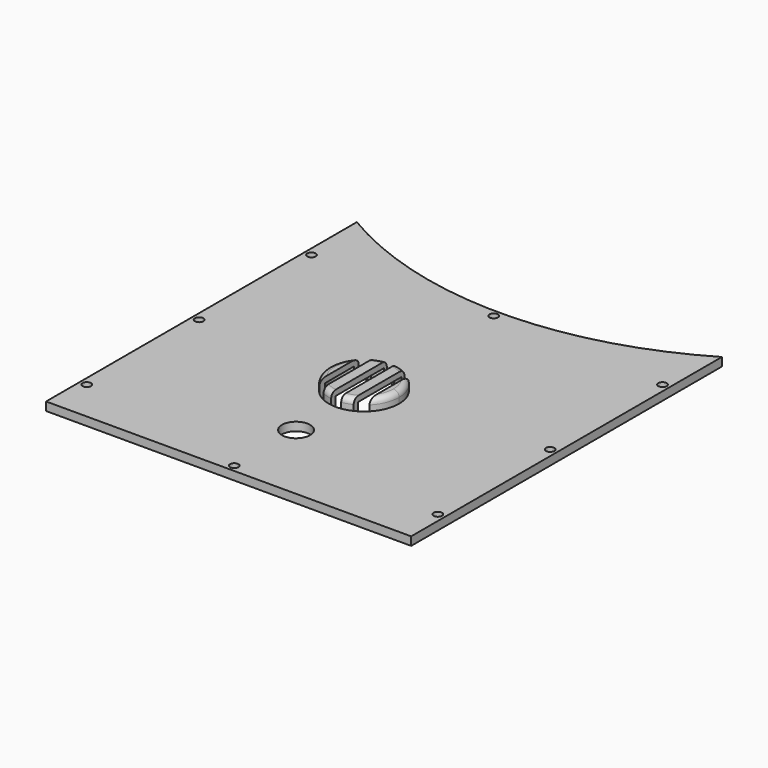
from build123d import *

# Parameters (mm, degrees)
F1_DEPTH  = 3
F2_R      = 1.5
F3_DEPTH  = 25
F5_DEPTH  = 4
F6_DEPTH  = 25
F7_R      = 2
F9_DEPTH  = 5
F10_R     = 5
F11_DEPTH = 25


# Not quite as in the source:
# - ends of sketch curves that miss each other by under 0.0002 mm in the source are joined


with BuildPart() as f1:
    # F0 (on Top) → F1 (new body)
    with BuildSketch(Plane.XY):
        with BuildLine():
            ThreePointArc((49.2280806434, 33.0130470502), (48.1713658013, 32.5621821126), (47.1108383201, 32.1203598507))
            Line((47.1108383201, 32.1203598507), (-4.1065374511, -22.3721440377))
            Line((-4.1065374511, -22.3721440377), (54.4172076095, -84.5927516487))
            Line((54.4172076095, -84.5927516487), (54.4172076095, 33.0130470502))
            Line((54.4172076095, 33.0130470502), (49.2280806434, 33.0130470502))
        make_face()
        Polygon((-4.1065374511, -22.3721440377), (-62.5827923905, -84.587700803), (-62.5827923905, -85.003347494), (54.4172076095, -85.003347494), (54.4172076095, -84.5927516487), align=None)
        with BuildLine():
            Line((-62.5827923905, 33.0130470502), (-62.5827923905, -84.587700803))
            Line((-62.5827923905, -84.587700803), (-4.1065374511, -22.3721440377))
            Line((-4.1065374511, -22.3721440377), (-55.4151337668, 32.1775440438))
            ThreePointArc((-55.4151337668, 32.1775440438), (-56.406067296, 32.5913463114), (-57.3936654243, 33.0130470502))
            Line((-57.3936654243, 33.0130470502), (-62.5827923905, 33.0130470502))
        make_face()
        with BuildLine():
            Line((-4.1065374511, -22.3721440377), (47.1108383201, 32.1203598507))
            ThreePointArc((47.1108383201, 32.1203598507), (-4.1578101896, 21.9966734267), (-55.4151337668, 32.1775440438))
            Line((-55.4151337668, 32.1775440438), (-4.1065374511, -22.3721440377))
        make_face()
        with BuildLine():
            ThreePointArc((60.9172316623, 46.8096119171), (-4.082778411, 28.996652506), (-69.0827923905, 46.8095976636))
            Line((-69.0827923905, 46.8095976636), (-69.0827923905, -91.503347494))
            Line((-69.0827923905, -91.503347494), (-62.5827923905, -84.587700803))
            Line((-62.5827923905, -84.587700803), (-62.5827923905, 33.0130470502))
            Line((-62.5827923905, 33.0130470502), (-57.3936654243, 33.0130470502))
            ThreePointArc((-57.3936654243, 33.0130470502), (-56.406067296, 32.5913463114), (-55.4151337668, 32.1775440438))
            ThreePointArc((-55.4151337668, 32.1775440438), (-4.1578101896, 21.9966734267), (47.1108383201, 32.1203598507))
            Line((47.1108383201, 32.1203598507), (60.9172316623, 46.8096119171))
        make_face()
        with BuildLine():
            Line((60.9172076095, -91.503347494), (60.9172076095, 46.809652506))
            Line((60.9172076095, 46.809652506), (47.1108383201, 32.1203598507))
            ThreePointArc((47.1108383201, 32.1203598507), (48.1713658013, 32.5621821126), (49.2280806434, 33.0130470502))
            Line((49.2280806434, 33.0130470502), (54.4172076095, 33.0130470502))
            Line((54.4172076095, 33.0130470502), (54.4172076095, -84.5927516487))
            Line((54.4172076095, -84.5927516487), (60.9172076095, -91.503347494))
        make_face()
        Polygon((-62.5827923905, -84.587700803), (-69.0827923905, -91.503347494), (60.9172076095, -91.503347494), (54.4172076095, -84.5927516487), (54.4172076095, -85.003347494), (-62.5827923905, -85.003347494), align=None)
    extrude(amount=F1_DEPTH)

    # F2 (on face) → F3 (cut)
    with BuildSketch(Plane.XY.offset(3)):
        with Locations((58.4172076095, -76.503347494)):
            Circle(F2_R)
        with Locations((58.4172076095, -26.503347494)):
            Circle(F2_R)
        with Locations((58.4172076095, 23.496652506)):
            Circle(F2_R)
        with Locations((-4.0827923905, 26.496652506)):
            Circle(F2_R)
        with Locations((-66.5827923905, -76.503347494)):
            Circle(F2_R)
        with Locations((-4.0827923905, -89.003347494)):
            Circle(F2_R)
        with Locations((-66.5827923905, -26.503347494)):
            Circle(F2_R)
        with Locations((-66.5827923905, 23.496652506)):
            Circle(F2_R)
    extrude(amount=-F3_DEPTH, mode=Mode.SUBTRACT)

    # F4 (on face) → F5 (join)
    with BuildSketch(Plane.XY.offset(3)):
        with BuildLine():
            Line((-13.011363819, -40.0015251468), (-13.011363819, -22.5051698412))
            ThreePointArc((-13.011363819, -22.5051698412), (-16.5827923905, -31.253347494), (-13.011363819, -40.0015251468))
        make_face()
        with BuildLine():
            ThreePointArc((4.8457790381, -40.0015251468), (7.4899588567, -35.9779034066), (8.4172076095, -31.253347494))
            ThreePointArc((8.4172076095, -31.253347494), (7.4899588567, -26.5287915814), (4.8457790381, -22.5051698412))
            Line((4.8457790381, -22.5051698412), (4.8457790381, -40.0015251468))
        make_face()
        with BuildLine():
            Line((1.2743504667, -42.5471962803), (1.2743504667, -19.9594987077))
            ThreePointArc((1.2743504667, -19.9594987077), (-0.4709241544, -19.2865430816), (-2.2970781048, -18.8815560114))
            Line((-2.2970781048, -18.8815560114), (-2.2970781048, -43.6251389767))
            ThreePointArc((-2.2970781048, -43.6251389767), (-0.4709241544, -43.2201519064), (1.2743504667, -42.5471962803))
        make_face()
        with BuildLine():
            Line((-5.8685066762, -43.6251389767), (-5.8685066762, -18.8815560114))
            ThreePointArc((-5.8685066762, -18.8815560114), (-7.6946606266, -19.2865430816), (-9.4399352476, -19.9594987077))
            Line((-9.4399352476, -19.9594987077), (-9.4399352476, -42.5471962803))
            ThreePointArc((-9.4399352476, -42.5471962803), (-7.6946606266, -43.2201519064), (-5.8685066762, -43.6251389767))
        make_face()
    extrude(amount=F5_DEPTH)

    # F4 (on face) → F6 (cut)
    with BuildSketch(Plane.XY.offset(3)):
        with BuildLine():
            Line((-9.4399352476, -42.5471962803), (-9.4399352476, -19.9594987077))
            ThreePointArc((-9.4399352476, -19.9594987077), (-11.3381709845, -21.0744732215), (-13.011363819, -22.5051698412))
            Line((-13.011363819, -22.5051698412), (-13.011363819, -40.0015251468))
            ThreePointArc((-13.011363819, -40.0015251468), (-11.3381709845, -41.4322217666), (-9.4399352476, -42.5471962803))
        make_face()
        with BuildLine():
            Line((-2.2970781048, -43.6251389767), (-2.2970781048, -18.8815560114))
            ThreePointArc((-2.2970781048, -18.8815560114), (-4.0827923905, -18.753347494), (-5.8685066762, -18.8815560114))
            Line((-5.8685066762, -18.8815560114), (-5.8685066762, -43.6251389767))
            ThreePointArc((-5.8685066762, -43.6251389767), (-4.0827923905, -43.753347494), (-2.2970781048, -43.6251389767))
        make_face()
        with BuildLine():
            Line((4.8457790381, -40.0015251468), (4.8457790381, -22.5051698412))
            ThreePointArc((4.8457790381, -22.5051698412), (3.1725862036, -21.0744732215), (1.2743504667, -19.9594987077))
            Line((1.2743504667, -19.9594987077), (1.2743504667, -42.5471962803))
            ThreePointArc((1.2743504667, -42.5471962803), (3.1725862036, -41.4322217666), (4.8457790381, -40.0015251468))
        make_face()
    extrude(amount=-F6_DEPTH, mode=Mode.SUBTRACT)

    # F7
    f7_edges = [f1.edges().sort_by_distance(p)[0] for p in [
        (-7.694661, -19.286543, 7),
        (-16.582792, -31.253347, 7),
        (-0.470924, -19.286543, 7),
        (8.417208, -31.253347, 7),
        (-0.470924, -43.220152, 7),
        (-7.694661, -43.220152, 7),
    ]]
    fillet(f7_edges, radius=F7_R)

    # F8 (on face) → F9 (cut)
    with BuildSketch(Plane(origin=(0, 0, 0), x_dir=(1, 0, 0), z_dir=(0, 0, -1))):
        with BuildLine():
            ThreePointArc((4.8457790381, 24.5226173164), (6.3865506098, 27.5722856522), (6.9172076095, 30.9476163238))
            ThreePointArc((6.9172076095, 30.9476163238), (6.3865506098, 34.3229469955), (4.8457790381, 37.3726153312))
            Line((4.8457790381, 37.3726153312), (4.8457790381, 24.5226173164))
        make_face()
        with BuildLine():
            Line((1.2743504667, 21.3402743185), (1.2743504667, 40.5549583292))
            ThreePointArc((1.2743504667, 40.5549583292), (-0.4573688452, 41.3330052967), (-2.2970781048, 41.8017042399))
            Line((-2.2970781048, 41.8017042399), (-2.2970781048, 20.0935284078))
            ThreePointArc((-2.2970781048, 20.0935284078), (-0.4573688452, 20.562227351), (1.2743504667, 21.3402743185))
        make_face()
        with BuildLine():
            Line((-2.2970781048, 20.0935284078), (-2.2970781048, 41.8017042399))
            ThreePointArc((-2.2970781048, 41.8017042399), (-4.0827923905, 41.9476163238), (-5.8685066762, 41.8017042399))
            Line((-5.8685066762, 41.8017042399), (-5.8685066762, 20.0935284078))
            ThreePointArc((-5.8685066762, 20.0935284078), (-4.0827923905, 19.9476163238), (-2.2970781048, 20.0935284078))
        make_face()
        with BuildLine():
            Line((-5.8685066762, 20.0935284078), (-5.8685066762, 41.8017042399))
            ThreePointArc((-5.8685066762, 41.8017042399), (-7.7082159357, 41.3330052967), (-9.4399352476, 40.5549583292))
            Line((-9.4399352476, 40.5549583292), (-9.4399352476, 21.3402743185))
            ThreePointArc((-9.4399352476, 21.3402743185), (-7.7082159357, 20.562227351), (-5.8685066762, 20.0935284078))
        make_face()
        with BuildLine():
            Line((-9.4399352476, 21.3402743185), (-9.4399352476, 40.5549583292))
            ThreePointArc((-9.4399352476, 40.5549583292), (-11.4007316429, 39.1602751562), (-13.011363819, 37.3726153312))
            Line((-13.011363819, 37.3726153312), (-13.011363819, 24.5226173164))
            ThreePointArc((-13.011363819, 24.5226173164), (-11.4007316429, 22.7349574914), (-9.4399352476, 21.3402743185))
        make_face()
        with BuildLine():
            Line((-13.011363819, 24.5226173164), (-13.011363819, 37.3726153312))
            ThreePointArc((-13.011363819, 37.3726153312), (-15.0827923905, 30.9476163238), (-13.011363819, 24.5226173164))
        make_face()
    extrude(amount=-F9_DEPTH, mode=Mode.SUBTRACT)

    # F10 (on face) → F11 (cut)
    with BuildSketch(Plane.XY.offset(3)):
        with Locations((-4.0827923905, -61.503347494)):
            Circle(F10_R)
    extrude(amount=-F11_DEPTH, mode=Mode.SUBTRACT)


solid = f1.part
